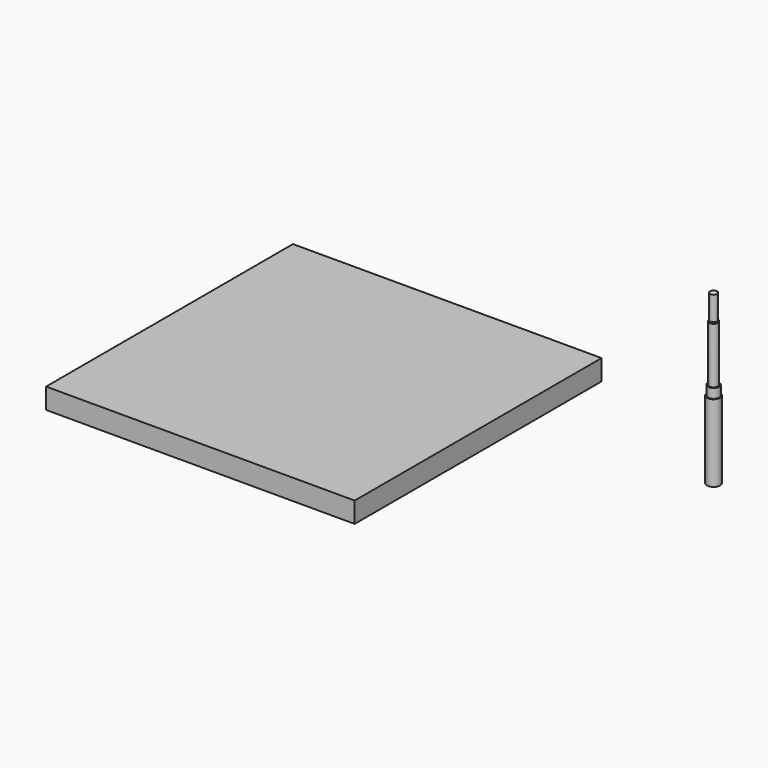
from build123d import *

# Parameters (mm, degrees)
F2_W     = 300
F2_H     = 300
F3_DEPTH = 20
F4_DEPTH = 13


# Not quite as in the source:
# - a feature names something its author has since deleted; it is built from what else it names


with BuildPart() as f1:
    # F0 (on Front) → F1 (revolve)
    with BuildSketch(Plane.XZ):
        Polygon((3.5, 108.6006758511), (0, 110.6006758511), (0, -41.3993241489), (6.35, -41.3993241489), (6.35, 20.6006758511), (5.5, 20.6006758511), (5.5, 29.8006758511), (4.3, 29.8006758511), (4.3, 84.1006758511), (3.5, 85.1006758511), align=None)
    revolve(axis=Axis((0, 0, 34.6006758511), (0, 0, -1)))

    # F4 (add): a face of the model
    f4_faces = [f1.faces().sort_by_distance(p)[0] for p in [
        (0, 0, -41.3993241489),
    ]]
    extrude(f4_faces, amount=F4_DEPTH)


with BuildPart() as f3:
    # F2 (on Top) → F3 (new body)
    with BuildSketch(Plane.XY):
        with Locations((-255.5129393935, -154.2015225627)):
            Rectangle(F2_W, F2_H)
    extrude(amount=F3_DEPTH)


solid = Compound([f1.part, f3.part])
